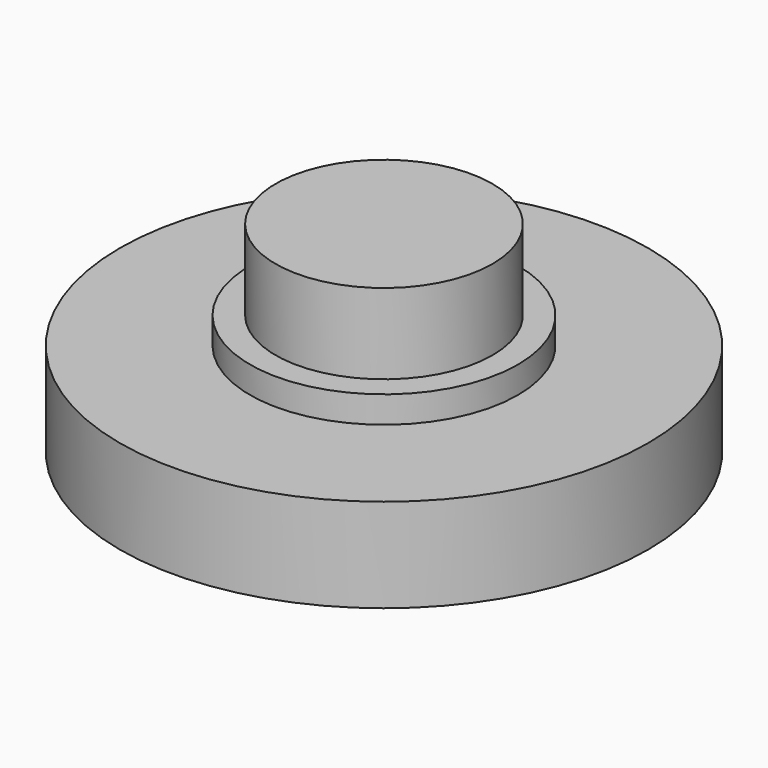
from build123d import *

# Parameters (mm, degrees)
F0_R     = 9.8592181747
F1_DEPTH = 3.5
F2_R     = 5
F3_DEPTH = 1
F4_R     = 4.05
F5_DEPTH = 3
F6_R     = 8.2811029309
F7_DEPTH = 1


# Not quite as in the source:
# - a fillet or chamfer that OpenCascade refuses, or shapes differently, is made with other operations: its cross-section is extruded or revolved along the edge and cut away or added


with BuildPart() as f1:
    # F0 (on Top) → F1 (new body)
    with BuildSketch(Plane.XY):
        Circle(F0_R)
    extrude(amount=F1_DEPTH)

    # F2 (on face) → F3 (join)
    with BuildSketch(Plane.XY.offset(3.5)):
        Circle(F2_R)
    extrude(amount=F3_DEPTH)

    # F4 (on face) → F5 (join)
    with BuildSketch(Plane.XY.offset(4.5)):
        Circle(F4_R)
    extrude(amount=F5_DEPTH)

    # F6 (on face) → F7 (cut)
    with BuildSketch(Plane(origin=(0, 0, 0), x_dir=(1, 0, 0), z_dir=(0, 0, -1))):
        Circle(F6_R)
    extrude(amount=-F7_DEPTH, mode=Mode.SUBTRACT)

    # F8: fillet of radius 32 on 1 edges, made by hand

    # F8_s1 → F8_t2 (revolve)
    with BuildSketch(Plane.XZ):
        with BuildLine():
            ThreePointArc((8.2811029309, 0), (4.3438489977, 0.7490157328), (0.3438489977, 1))
            Line((0.3438489977, 1), (8.2811029309, 1))
            Line((8.2811029309, 1), (8.2811029309, 0))
        make_face()
    revolve(axis=Axis((0, 0, 1), (0, 0, -1)))


solid = f1.part
